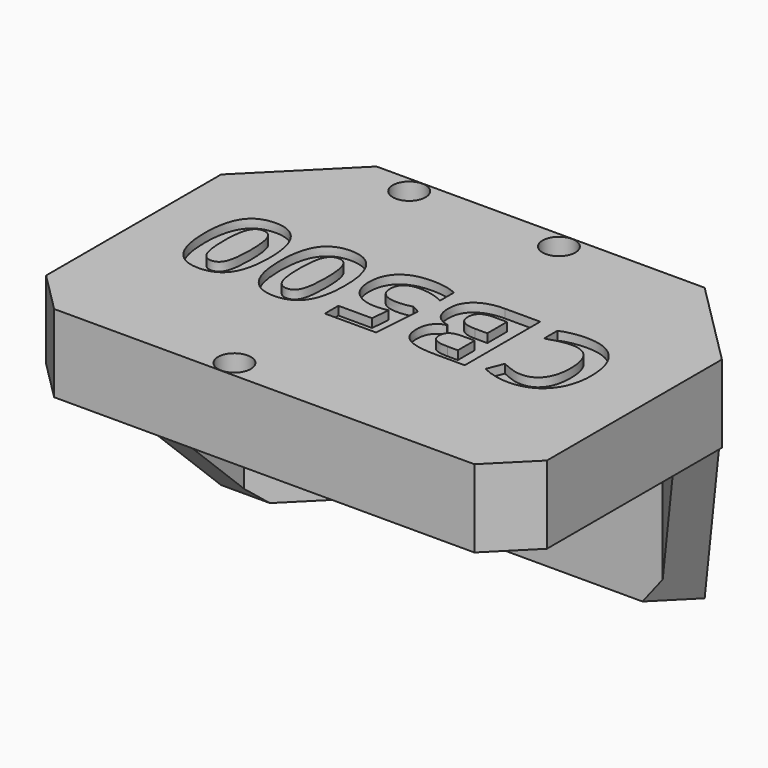
from build123d import *

# Parameters (mm, degrees)
F1_DEPTH      = 13.5
F2_T          = -6
F4_DEPTH      = 34
F6_R          = 1.6
F7_DEPTH      = 60
F9_DEPTH      = 8.4862813742
F10_R         = 2.85
F11_DEPTH     = 3.2
F12_TEXT_SIZE = 22.9461175989
F13_DEPTH     = 1.5
F15_DEPTH     = 8.4862813742
F16_W         = 52.0294372515
F16_H         = 7.5
F17_DEPTH     = 1
F18_W         = 68.0294372515
F18_H         = 7.5
F19_DEPTH     = 1


# Not quite as in the source:
# - Text() gives the source's letters only with a copy of the font that has no kerning and outlines rounded to 1/6400 em; it was checked with that copy


with BuildPart() as f1:
    # F0 (on Top) → F1 (new body)
    with BuildSketch(Plane.XY):
        Polygon((-87, 45), (-87, 7), (-80, 0), (-7, 0), (0, 7), (0, 45), (-15, 60), (-72, 60), align=None)
    extrude(amount=F1_DEPTH)

    # F2
    f2_openings = [f1.faces().sort_by_distance(p)[0] for p in [
        (-43.5, 29.136811, 0),
    ]]
    offset(amount=F2_T, openings=f2_openings)

    # F3 (on face) → F4 (join)
    with BuildSketch(Plane(origin=(0, 0, 0), x_dir=(1, 0, 0), z_dir=(0, 0, -1))):
        Polygon((-81, -42.5147186258), (-81, -9.4852813742), (-87, -9.4852813742), (-87, -45), (-72, -60), (-15, -60), (-1.7573593129, -46.7573593129), (-6, -42.5147186258), (-17.4852813742, -54), (-69.5147186258, -54), align=None)
    extrude(amount=F4_DEPTH)

    # F6 (on face) → F7 (cut)
    with BuildSketch(Plane.XY.offset(13.5)):
        with Locations((-38, 57.1)):
            Circle(F6_R)
        with Locations((-64, 57.1)):
            Circle(F6_R)
        with Locations((-51, 2.9)):
            Circle(F6_R)
    extrude(amount=-F7_DEPTH, mode=Mode.SUBTRACT)

    # F8 (on face) → F9 (cut, through all)
    with BuildSketch(Plane(origin=(-87, 0, 0), x_dir=(0, -1, 0), z_dir=(-1, 0, 0))):
        Polygon((-9.4852813742, -34), (-9.4852813742, 0), (-45, -34), align=None)
    extrude(amount=-F9_DEPTH, mode=Mode.SUBTRACT)

    # F10 (on face) → F11 (cut)
    with BuildSketch(Plane.XY.offset(13.5)):
        with Locations((-64, 57.1)):
            Circle(F10_R)
        with Locations((-38, 57.1)):
            Circle(F10_R)
        with Locations((-51, 2.9)):
            Circle(F10_R)
    extrude(amount=-F11_DEPTH, mode=Mode.SUBTRACT)

    # F12 (on face) → F13 (cut)
    with BuildSketch(Plane.XY.offset(13.5)):
        with Locations(Location((-9.5, 38.27), (0, 0, -180))):
            Text('CB500', F12_TEXT_SIZE, font='Open Sans', font_style=FontStyle.BOLD, text_align=(TextAlign.LEFT, TextAlign.BOTTOM))
    extrude(amount=-F13_DEPTH, mode=Mode.SUBTRACT)

    # F14 (on face) → F15 (cut, through all)
    with BuildSketch(Plane(origin=(22.5, 22.5, 0), x_dir=(-0.7071067812, 0.7071067812, 0), z_dir=(0.7071067812, 0.7071067812, 0))):
        Polygon((53.033008589, -34), (34.3050865276, 0), (31.8198051534, 0), (31.8198051534, -34), align=None)
    extrude(amount=-F15_DEPTH, mode=Mode.SUBTRACT)

    # F16 (on face) → F17 (join)
    with BuildSketch(Plane.XZ.offset(-54)):
        with Locations((-43.5, 3.75)):
            Rectangle(F16_W, F16_H)
    extrude(amount=F17_DEPTH)

    # F18 (on face) → F19 (join)
    with BuildSketch(Plane(origin=(0, 6, 0), x_dir=(-1, 0, 0), z_dir=(0, 1, 0))):
        with Locations((43.5, 3.75)):
            Rectangle(F18_W, F18_H)
    extrude(amount=F19_DEPTH)


solid = f1.part
